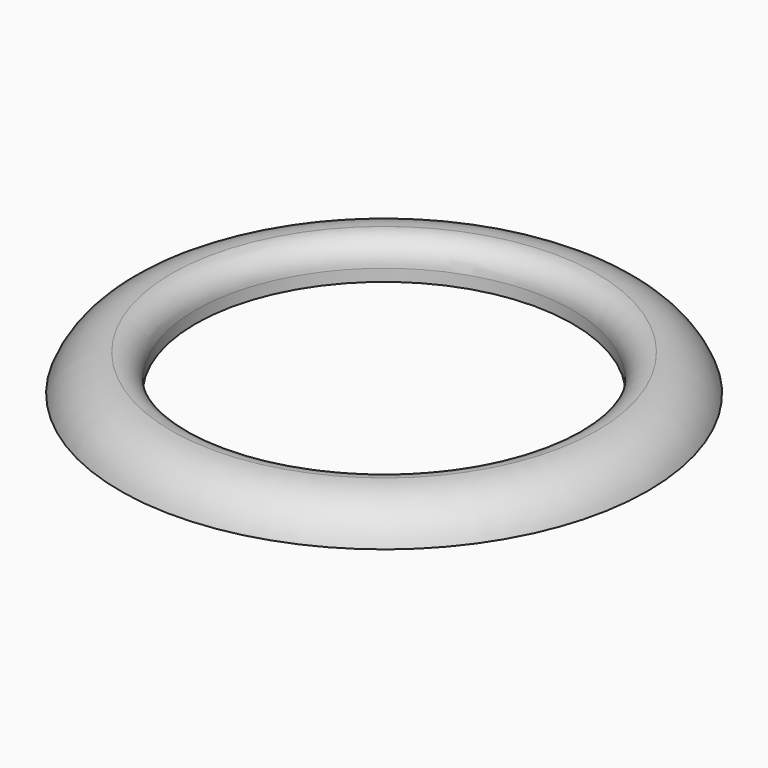
from build123d import *

# Parameters (mm, degrees)
F0_R     = 11.1125
F0_R_2   = 7.9375
F1_DEPTH = 1.524
F3_R     = 1.016


# Not quite as in the source:
# - a fillet or chamfer that OpenCascade refuses, or shapes differently, is made with other operations: its cross-section is extruded or revolved along the edge and cut away or added


with BuildPart() as f1:
    # F0 (on Top) → F1 (new body)
    with BuildSketch(Plane.XY):
        Circle(F0_R)
        Circle(F0_R_2, mode=Mode.SUBTRACT)
    extrude(amount=F1_DEPTH)

    # F2: fillet of radius 2.286 on 1 edges, made by hand

    # F2_s1 → F2_t2 (revolve, cut)
    with BuildSketch(Plane.XZ):
        with BuildLine():
            ThreePointArc((11.1125, 0), (10.2770612463, 1.104511184), (8.9572385309, 1.524))
            Line((8.9572385309, 1.524), (11.1125, 1.524))
            Line((11.1125, 1.524), (11.1125, 0))
        make_face()
    revolve(axis=Axis((0, 0, 1.524), (0, 0, 1)), mode=Mode.SUBTRACT)

    # F3
    f3_edges = [f1.edges().sort_by_distance(p)[0] for p in [
        (-7.9375, 0, 1.524),
    ]]
    fillet(f3_edges, radius=F3_R)


solid = f1.part
